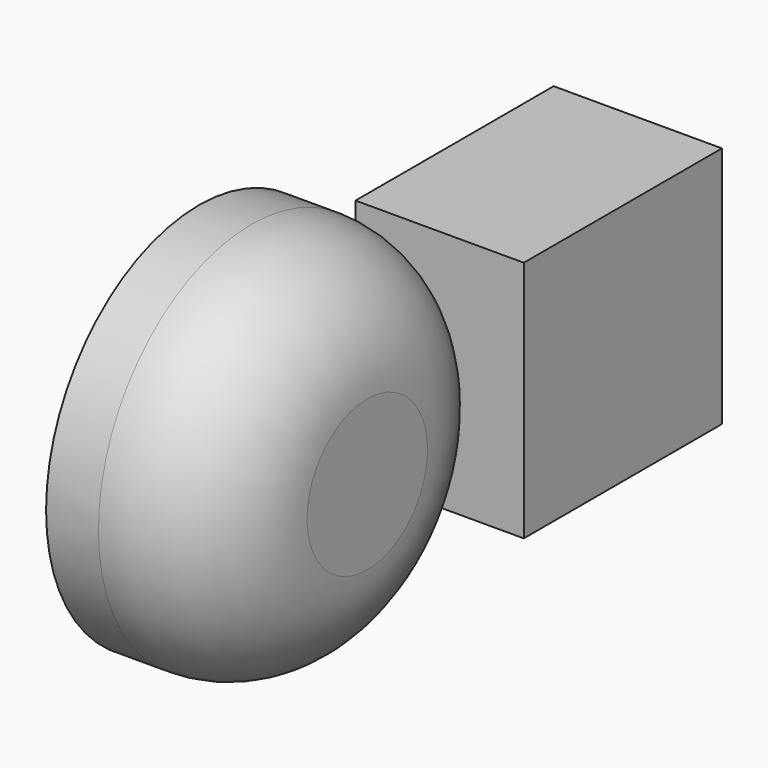
from build123d import *

# Parameters (mm, degrees)
F0_R     = 30.4208936765
F1_DEPTH = 26.77935
F0_W     = 39.4137930125
F0_H     = 38.6255178601
F2_R     = 18.4450744592


# Not quite as in the source:
# - the program builds the solid bodies; features that only make, move or delete a surface that nothing else refers to are left out


with BuildPart() as f1:
    # F0 (on Right) → F1 (new body)
    with BuildSketch(Plane.YZ):
        Circle(F0_R)
    extrude(amount=F1_DEPTH)

    # F2
    f2_edges = [f1.edges().sort_by_distance(p)[0] for p in [
        (26.77935, -30.420894, 0),
    ]]
    fillet(f2_edges, radius=F2_R)


with BuildPart() as f1b:
    # F0 (on Right) → F1, piece 2 (new body)
    with BuildSketch(Plane.YZ):
        with Locations((50.8410567418, -0.9196558967)):
            Rectangle(F0_W, F0_H)
    extrude(amount=F1_DEPTH)


solid = Compound([f1.part, f1b.part])
